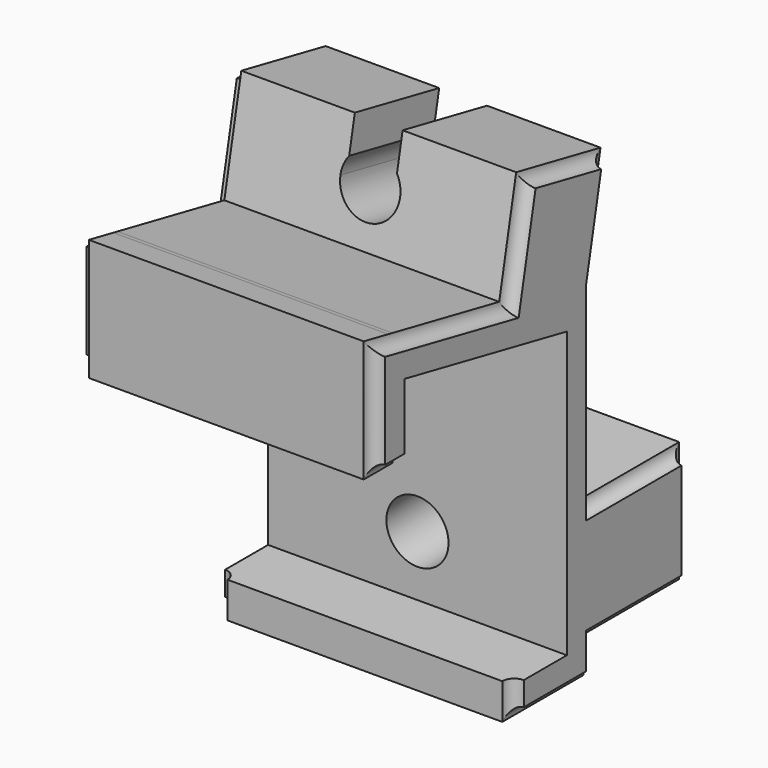
from build123d import *

# Parameters (mm, degrees)
F0_W      = 10
F0_H      = 10.1
F1_DEPTH  = 25
F3_DEPTH  = 24.6375403377
F4_R      = 2.6
F5_DEPTH  = 33.001
F7_DEPTH  = 1
F9_DEPTH  = 1
F11_DEPTH = 1
F12_R     = 0.99999
F13_R     = 0.99999


# Not quite as in the source:
# - a fillet or chamfer is up to 0.001 mm smaller than in the source, because OpenCascade refuses the exact size


with BuildPart() as f1:
    # F0 (on Right) → F1 (new body)
    with BuildSketch(Plane.YZ):
        Polygon((8.7376843859, -5.3593200147), (3.235891927, -5.3593200147), (3.235891927, -8.3593200147), (8.7376843859, -8.3593200147), (11.7376843859, -8.3593200147), (11.7376843859, -5.3593200147), (11.7376843859, 4.7406799853), (11.7376843859, 20.9479271312), (2.9139854062, 22.7205907531), (-8.2623156141, 24.9658874581), (-8.2623156141, 21.9059462631), (-5.6975004546, 21.3906799853), (8.7376843859, 18.4906799853), align=None)
        Polygon((-8.2623156141, 15.3906799853), (-8.2623156141, 21.9059462631), (-8.2623156141, 24.9658874581), (-8.6975004546, 25.0533152293), (-11.2623156141, 25.5685815071), (-11.2623156141, 15.3906799853), (-8.6975004546, 15.3906799853), align=None)
        with Locations((16.7376843859, -0.3093200147)):
            Rectangle(F0_W, F0_H)
        Polygon((4.6866490281, 31.5442897327), (2.9139854062, 22.7205907531), (11.7376843859, 20.9479271312), (13.5103480077, 29.7716261109), align=None)
    extrude(amount=F1_DEPTH)

    # F2 (on face) → F3 (cut, through all)
    with BuildSketch(Plane(origin=(0, 7.2371941298, -1.4539379446), x_dir=(-1, 0, 0), z_dir=(0, 0.9804109977, -0.1969626246))):
        with BuildLine():
            ThreePointArc((-14.5, 28.8494632633), (-13.290569415, 24.9777550181), (-10, 27.3494632633))
            ThreePointArc((-10, 27.3494632633), (-10.1282917549, 28.1400326783), (-10.5, 28.8494632633))
            ThreePointArc((-10.5, 28.8494632633), (-12.5, 29.8494632633), (-14.5, 28.8494632633))
        make_face()
        with BuildLine():
            ThreePointArc((-14.5, 28.8494632633), (-12.5, 29.8494632633), (-10.5, 28.8494632633))
            Line((-10.5, 28.8494632633), (-10.5, 31.8494632633))
            Line((-10.5, 31.8494632633), (-12.5, 31.8494632633))
            Line((-12.5, 31.8494632633), (-14.5, 31.8494632633))
            Line((-14.5, 31.8494632633), (-14.5, 28.8494632633))
        make_face()
    extrude(amount=-F3_DEPTH, mode=Mode.SUBTRACT)

    # F4 (on face) → F5 (cut, through all)
    with BuildSketch(Plane(origin=(0, 21.7376843859, 0), x_dir=(-1, 0, 0), z_dir=(0, 1, 0))):
        with Locations((-12.5, -0.3093200147)):
            Circle(F4_R)
    extrude(amount=-F5_DEPTH, mode=Mode.SUBTRACT)

    # F6 (on face) → F7 (cut)
    with BuildSketch(Plane(origin=(0, 0, 0), x_dir=(0, -1, 0), z_dir=(-1, 0, 0))):
        Polygon((0.6576159399, 20.3781771837), (8.2623156141, 15.3906799853), (8.2623156141, 21.9059462631), align=None)
    extrude(amount=-F7_DEPTH, mode=Mode.SUBTRACT)

    # F8 (on face) → F9 (cut)
    with BuildSketch(Plane.YZ.offset(25)):
        Polygon((-11.2623156141, 15.3906799853), (-8.2623156141, 15.3906799853), (-8.2623156141, 16.3906799853), (-10.2623156141, 16.3906799853), (-10.2623156141, 24.3477030924), (3.6974337793, 21.5432171307), (5.4700974012, 30.3669161103), (12.3329743853, 28.9881777378), (10.7376843859, 21.0473825599), (10.7376843859, 3.7406799853), (20.7376843859, 3.7406799853), (20.7376843859, -4.3593200147), (10.7376843859, -4.3593200147), (10.7376843859, -7.3593200147), (4.235891927, -7.3593200147), (4.235891927, -5.3593200147), (3.235891927, -5.3593200147), (3.235891927, -8.3593200147), (11.7376843859, -8.3593200147), (11.7376843859, -5.3593200147), (21.7376843859, -5.3593200147), (21.7376843859, 4.7406799853), (11.7376843859, 4.7406799853), (11.7376843859, 20.9479271312), (13.5103480077, 29.7716261109), (4.6866490281, 31.5442897327), (2.9139854062, 22.7205907531), (-11.2623156141, 25.5685815071), align=None)
    extrude(amount=-F9_DEPTH, mode=Mode.SUBTRACT)

    # F10 (on face) → F11 (cut)
    with BuildSketch(Plane(origin=(0, 0, 0), x_dir=(0, -1, 0), z_dir=(-1, 0, 0))):
        Polygon((8.2623156141, 16.3906799853), (8.2623156141, 15.3906799853), (11.2623156141, 15.3906799853), (11.2623156141, 25.5685815071), (-2.9139854062, 22.7205907531), (-4.6866490281, 31.5442897327), (-13.5103480077, 29.7716261109), (-11.7376843859, 20.9479271312), (-11.7376843859, 4.7406799853), (-21.7376843859, 4.7406799853), (-21.7376843859, -5.3593200147), (-11.7376843859, -5.3593200147), (-11.7376843859, -8.3593200147), (-3.235891927, -8.3593200147), (-3.235891927, -5.3593200147), (-4.235891927, -5.3593200147), (-4.235891927, -7.3593200147), (-10.7376843859, -7.3593200147), (-10.7376843859, -4.3593200147), (-20.7376843859, -4.3593200147), (-20.7376843859, 3.7406799853), (-10.7376843859, 3.7406799853), (-10.7376843859, 21.0473825599), (-12.3329743853, 28.9881777378), (-5.4700974012, 30.3669161103), (-3.6974337793, 21.5432171307), (10.2623156141, 24.3477030924), (10.2623156141, 16.3906799853), align=None)
    extrude(amount=-F11_DEPTH, mode=Mode.SUBTRACT)

    # F12 (radius 1 in the source; OpenCascade refuses exactly that, so slightly less here)
    f12_edges = [f1.edges().sort_by_distance(p)[0] for p in [
        (24, 4.235892, -6.35932),
        (24, 7.486788, -7.35932),
        (24, 15.737684, -4.35932),
        (24, 10.737684, -5.85932),
        (24, 20.737684, -0.30932),
        (24, 10.737684, 12.394031),
        (24, 15.737684, 3.74068),
        (24, 11.535329, 25.01778),
        (24, 8.901536, 29.677547),
        (24, -3.282441, 22.94546),
        (24, 4.583766, 25.955067),
        (24, -10.262316, 20.369192),
        (24, -9.262316, 16.39068),
    ]]
    fillet(f12_edges, radius=F12_R)

    # F13 (radius 1 in the source; OpenCascade refuses exactly that, so slightly less here)
    f13_edges = [f1.edges().sort_by_distance(p)[0] for p in [
        (1, 4.235892, -6.35932),
        (1, 7.486788, -7.35932),
        (1, 15.737684, -4.35932),
        (1, 10.737684, -5.85932),
        (1, 20.737684, -0.30932),
        (1, 10.737684, 12.394031),
        (1, 15.737684, 3.74068),
        (1, 11.535329, 25.01778),
        (1, 8.901536, 29.677547),
        (1, -3.282441, 22.94546),
        (1, 4.583766, 25.955067),
        (1, -10.262316, 20.369192),
        (1, -9.262316, 16.39068),
    ]]
    fillet(f13_edges, radius=F13_R)


solid = f1.part
